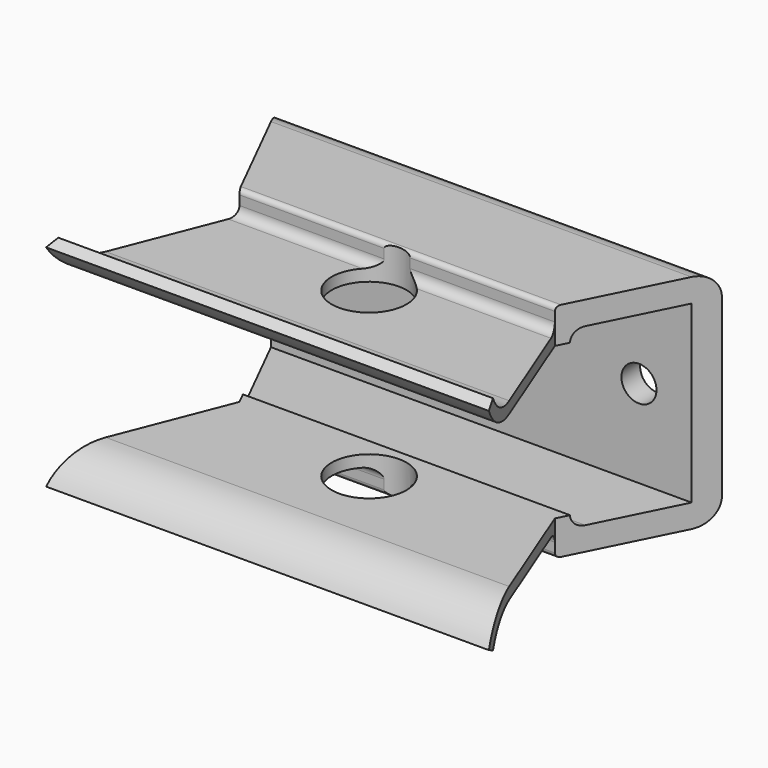
from build123d import *

# Parameters (mm, degrees)
F0_R     = 16
F1_DEPTH = 47.5
F3_DEPTH = 95
F5_D     = 15


# Not quite as in the source:
# - ends of sketch curves that miss each other by under 0.0002 mm in the source are joined


with BuildPart() as f1:
    # F0 (on Top) → F1 (new body, symmetric)
    with BuildSketch(Plane.XY):
        Polygon((95, 0), (0, 0), (-95, 0), (-67.5, -55), (-95, -125), (0, -125), (95, -125), (67.5, -55), align=None)
        with Locations((0, -70)):
            Circle(F0_R, mode=Mode.SUBTRACT)
    extrude(amount=F1_DEPTH, both=True)

    # F2 (on Right) → F3 (intersect, symmetric)
    with BuildSketch(Plane.YZ):
        with BuildLine():
            Line((-10, 0), (0, 0))
            Line((0, 0), (0, 37.5))
            ThreePointArc((0, 37.5), (-2.9289321881, 44.5710678119), (-10, 47.5))
            Line((-10, 47.5), (-53, 47.5))
            ThreePointArc((-53, 47.5), (-54.4142135624, 46.9142135624), (-55, 45.5))
            Line((-55, 45.5), (-55, 41.5))
            ThreePointArc((-55, 41.5), (-56.1715728753, 38.6715728753), (-59, 37.5))
            Line((-59, 37.5), (-103, 37.5))
            ThreePointArc((-103, 37.5), (-112.8615414617, 40.1853795152), (-120, 47.5))
            Line((-120, 47.5), (-124.3701794471, 45.0706943661))
            ThreePointArc((-124.3701794471, 45.0706943661), (-115.3966418036, 35.8757089339), (-103, 32.5000005737))
            Line((-103, 32.5000005737), (-50, 32.5000005737))
            ThreePointArc((-50, 32.5000005737), (-48.5355339059, 36.0355339059), (-45, 37.5))
            Line((-45, 37.5), (-10, 37.5))
            Line((-10, 37.5), (-10, 0))
        make_face()
        with BuildLine():
            Line((0, -37.5), (0, 0))
            Line((0, 0), (-10, 0))
            Line((-10, 0), (-10, -37.5))
            Line((-10, -37.5), (-45, -37.5))
            ThreePointArc((-45, -37.5), (-48.5355339059, -36.0355339059), (-50, -32.5))
            Line((-50, -32.5), (-103, -32.5000005737))
            ThreePointArc((-103, -32.5000005737), (-115.3966418036, -35.8757089339), (-124.3701794471, -45.0706943661))
            Line((-124.3701794471, -45.0706943661), (-120, -47.5))
            ThreePointArc((-120, -47.5), (-112.8615414617, -40.1853795152), (-103, -37.5))
            Line((-103, -37.5), (-59, -37.5))
            ThreePointArc((-59, -37.5), (-56.1715728753, -38.6715728753), (-55, -41.5))
            Line((-55, -41.5), (-55, -45.5))
            ThreePointArc((-55, -45.5), (-54.4142135624, -46.9142135624), (-53, -47.5))
            Line((-53, -47.5), (-10, -47.5))
            ThreePointArc((-10, -47.5), (-2.9289321881, -44.5710678119), (0, -37.5))
        make_face()
    extrude(amount=F3_DEPTH, both=True, mode=Mode.INTERSECT)

    # F5 (through all)
    with Locations(Plane(origin=(0, 0, 0), x_dir=(-1, 0, 0), z_dir=(0, 1, 0))):
        with Locations((67.5, 0), (-67.5, 0)):
            Hole(F5_D / 2)


solid = f1.part
